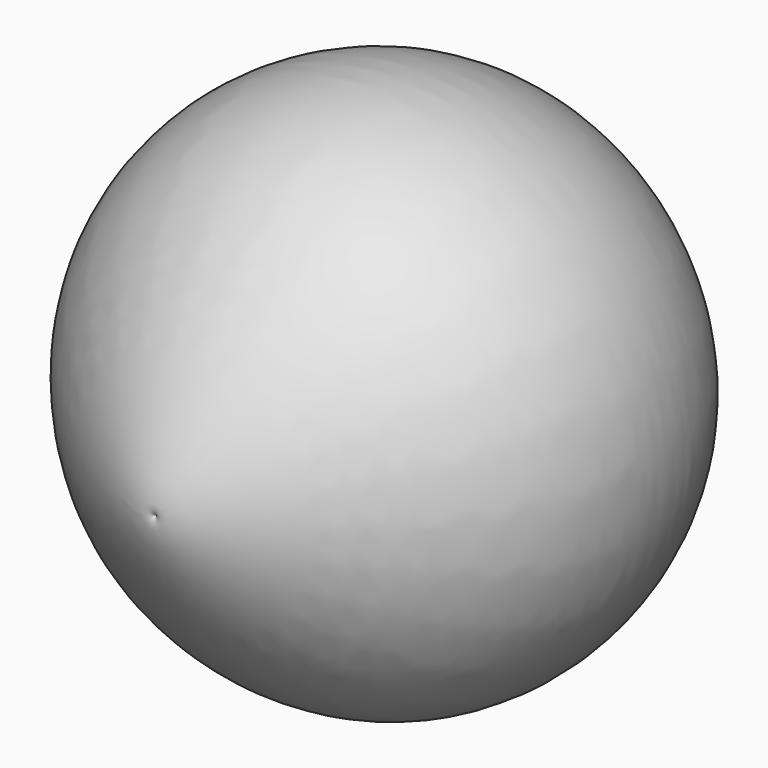
from build123d import *


with BuildPart() as f0:
    # F1 (on Top) → F0 (revolve)
    with BuildSketch(Plane.XY):
        with BuildLine():
            add(Edge.make_bspline(
                [(0, -75.5448117852), (-1.8620630786, -81.250339653), (-77.8677379206, -43.4844162391), (-60.6429222345, 36.5103540419), (-24.3347199185, 48.3725431206), (-23.6140117049, 45.2670753002)],
                knots=[0.4286973187, 0.4286973187, 0.4286973187, 0.4286973187, 0.6406510243, 0.8641701403, 1, 1, 1, 1], degree=3))
            Line((0, -75.5448117852), (0, -74.3976985995))
            add(Edge.make_bspline(
                [(-23.6140117049, 45.2670753002), (-22.6363500957, 41.0544180698), (-74.5912576464, -0.0964419028), (-1.9818544789, -65.3230744632), (0, -74.3976985995)],
                knots=[0, 0, 0, 0, 0.1842571469, 0.4171126423, 0.4171126423, 0.4171126423, 0.4171126423], degree=3))
        make_face()
    revolve(axis=Axis((0, -26.8867425621, 0), (0, 1, 0)))


solid = f0.part
